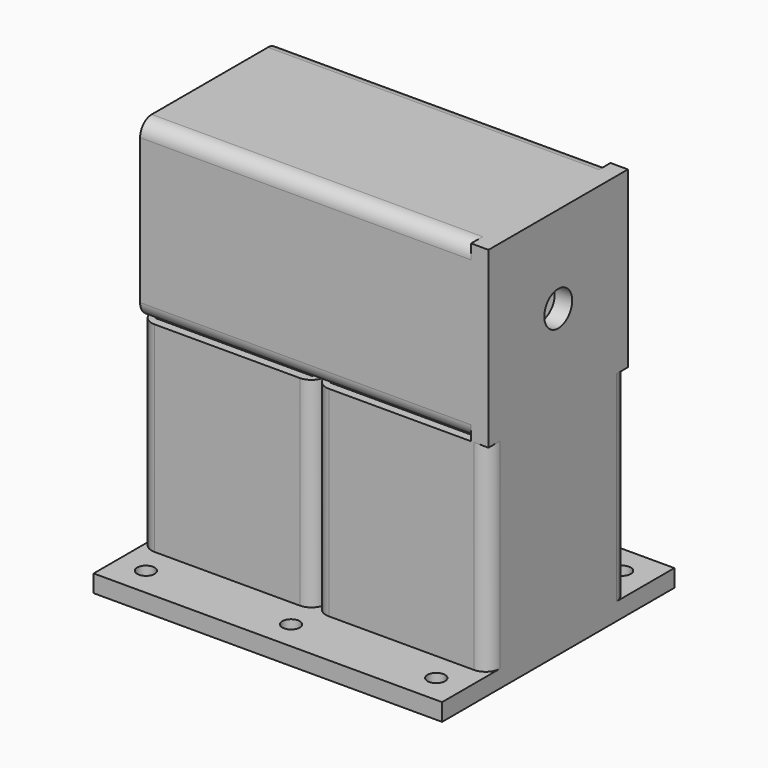
from build123d import *

# Parameters (mm, degrees)
F0_W     = 54
F0_H     = 54
F1_DEPTH = 69
F2_R     = 3
F2_W     = 54
F2_H     = 54
F3_DEPTH = 6
F4_W     = 54
F4_H     = 54
F5_DEPTH = 120
F6_W     = 60
F6_H     = 60
F6_R     = 6
F7_DEPTH = 6


with BuildPart() as f1:
    # F0 (on Top) → F1 (new body)
    with BuildSketch(Plane.XY):
        with BuildLine():
            ThreePointArc((-5.85040465, -3.5986092687), (-9.3859385559, -5.0630753627), (-10.85040465, -8.5986092687))
            Line((-10.85040465, -8.5986092687), (-10.85040465, -58.5986092687))
            ThreePointArc((-10.85040465, -58.5986092687), (-9.3859385559, -62.1341431746), (-5.85040465, -63.5986092687))
            Line((-5.85040465, -63.5986092687), (44.14959535, -63.5986092687))
            ThreePointArc((44.14959535, -63.5986092687), (47.685129256, -62.1341431746), (49.14959535, -58.5986092687))
            Line((49.14959535, -58.5986092687), (49.14959535, -8.5986092687))
            ThreePointArc((49.14959535, -8.5986092687), (47.685129256, -5.0630753627), (44.14959535, -3.5986092687))
            Line((44.14959535, -3.5986092687), (-5.85040465, -3.5986092687))
        make_face()
        with Locations((19.14959535, -33.5986092687)):
            Rectangle(F0_W, F0_H, mode=Mode.SUBTRACT)
        with BuildLine():
            ThreePointArc((54.14959535, -3.5986092687), (50.6140614441, -5.0630753627), (49.14959535, -8.5986092687))
            Line((49.14959535, -8.5986092687), (49.14959535, -58.5986092687))
            ThreePointArc((49.14959535, -58.5986092687), (50.6140614441, -62.1341431746), (54.14959535, -63.5986092687))
            Line((54.14959535, -63.5986092687), (104.14959535, -63.5986092687))
            ThreePointArc((104.14959535, -63.5986092687), (107.685129256, -62.1341431746), (109.14959535, -58.5986092687))
            Line((109.14959535, -58.5986092687), (109.14959535, -8.5986092687))
            ThreePointArc((109.14959535, -8.5986092687), (107.685129256, -5.0630753627), (104.14959535, -3.5986092687))
            Line((104.14959535, -3.5986092687), (54.14959535, -3.5986092687))
        make_face()
        with Locations((79.14959535, -33.5986092687)):
            Rectangle(F0_W, F0_H, mode=Mode.SUBTRACT)
    extrude(amount=F1_DEPTH)

    # F2 (on face) → F3 (join)
    with BuildSketch(Plane(origin=(0, 0, 0), x_dir=(1, 0, 0), z_dir=(0, 0, -1))):
        with BuildLine():
            Line((-10.85040465, -16.4013907313), (109.14959535, -16.4013907313))
            Line((109.14959535, -16.4013907313), (109.14959535, 8.5986092687))
            ThreePointArc((109.14959535, 8.5986092687), (107.685129256, 5.0630753627), (104.14959535, 3.5986092687))
            Line((104.14959535, 3.5986092687), (54.14959535, 3.5986092687))
            ThreePointArc((54.14959535, 3.5986092687), (50.6140614441, 5.0630753627), (49.14959535, 8.5986092687))
            ThreePointArc((49.14959535, 8.5986092687), (47.685129256, 5.0630753627), (44.14959535, 3.5986092687))
            Line((44.14959535, 3.5986092687), (-5.85040465, 3.5986092687))
            ThreePointArc((-5.85040465, 3.5986092687), (-9.3859385559, 5.0630753627), (-10.85040465, 8.5986092687))
            Line((-10.85040465, 8.5986092687), (-10.85040465, -16.4013907313))
        make_face()
        with Locations((-0.85040465, -6.4013907313)):
            Circle(F2_R, mode=Mode.SUBTRACT)
        with Locations((49.14959535, -6.4013907313)):
            Circle(F2_R, mode=Mode.SUBTRACT)
        with Locations((99.14959535, -6.4013907313)):
            Circle(F2_R, mode=Mode.SUBTRACT)
        with BuildLine():
            ThreePointArc((104.14959535, 63.5986092687), (107.685129256, 62.1341431746), (109.14959535, 58.5986092687))
            Line((109.14959535, 58.5986092687), (109.14959535, 83.5986092687))
            Line((109.14959535, 83.5986092687), (-10.85040465, 83.5986092687))
            Line((-10.85040465, 83.5986092687), (-10.85040465, 58.5986092687))
            ThreePointArc((-10.85040465, 58.5986092687), (-9.3859385559, 62.1341431746), (-5.85040465, 63.5986092687))
            Line((-5.85040465, 63.5986092687), (44.14959535, 63.5986092687))
            ThreePointArc((44.14959535, 63.5986092687), (47.685129256, 62.1341431746), (49.14959535, 58.5986092687))
            ThreePointArc((49.14959535, 58.5986092687), (50.6140614441, 62.1341431746), (54.14959535, 63.5986092687))
            Line((54.14959535, 63.5986092687), (104.14959535, 63.5986092687))
        make_face()
        with Locations((-0.85040465, 73.5986092687)):
            Circle(F2_R, mode=Mode.SUBTRACT)
        with Locations((49.14959535, 73.5986092687)):
            Circle(F2_R, mode=Mode.SUBTRACT)
        with Locations((99.14959535, 73.5986092687)):
            Circle(F2_R, mode=Mode.SUBTRACT)
        with BuildLine():
            ThreePointArc((104.14959535, 3.5986092687), (107.685129256, 5.0630753627), (109.14959535, 8.5986092687))
            Line((109.14959535, 8.5986092687), (109.14959535, 58.5986092687))
            ThreePointArc((109.14959535, 58.5986092687), (107.685129256, 62.1341431746), (104.14959535, 63.5986092687))
            Line((104.14959535, 63.5986092687), (54.14959535, 63.5986092687))
            ThreePointArc((54.14959535, 63.5986092687), (50.6140614441, 62.1341431746), (49.14959535, 58.5986092687))
            ThreePointArc((49.14959535, 58.5986092687), (47.685129256, 62.1341431746), (44.14959535, 63.5986092687))
            Line((44.14959535, 63.5986092687), (-5.85040465, 63.5986092687))
            ThreePointArc((-5.85040465, 63.5986092687), (-9.3859385559, 62.1341431746), (-10.85040465, 58.5986092687))
            Line((-10.85040465, 58.5986092687), (-10.85040465, 8.5986092687))
            ThreePointArc((-10.85040465, 8.5986092687), (-9.3859385559, 5.0630753627), (-5.85040465, 3.5986092687))
            Line((-5.85040465, 3.5986092687), (44.14959535, 3.5986092687))
            ThreePointArc((44.14959535, 3.5986092687), (47.685129256, 5.0630753627), (49.14959535, 8.5986092687))
            ThreePointArc((49.14959535, 8.5986092687), (50.6140614441, 5.0630753627), (54.14959535, 3.5986092687))
            Line((54.14959535, 3.5986092687), (104.14959535, 3.5986092687))
        make_face()
        with Locations((19.14959535, 33.5986092687)):
            Rectangle(F2_W, F2_H, mode=Mode.SUBTRACT)
        with Locations((79.14959535, 33.5986092687)):
            Rectangle(F2_W, F2_H, mode=Mode.SUBTRACT)
        with Locations((19.14959535, 33.5986092687)):
            Rectangle(F2_W, F2_H)
        with Locations((79.14959535, 33.5986092687)):
            Rectangle(F2_W, F2_H)
    extrude(amount=F3_DEPTH)

    # F4 (on face) → F5 (join, through all)
    with BuildSketch(Plane.YZ.offset(109.14959535)):
        with BuildLine():
            ThreePointArc((-3.5986092687, 124), (-5.0630753627, 127.5355339059), (-8.5986092687, 129))
            Line((-8.5986092687, 129), (-58.5986092687, 129))
            ThreePointArc((-58.5986092687, 129), (-62.1341431746, 127.5355339059), (-63.5986092687, 124))
            Line((-63.5986092687, 124), (-63.5986092687, 74))
            ThreePointArc((-63.5986092687, 74), (-62.1341431746, 70.4644660941), (-58.5986092687, 69))
            Line((-58.5986092687, 69), (-8.5986092687, 69))
            ThreePointArc((-8.5986092687, 69), (-5.0630753627, 70.4644660941), (-3.5986092687, 74))
            Line((-3.5986092687, 74), (-3.5986092687, 124))
        make_face()
        with Locations((-33.5986092687, 99)):
            Rectangle(F4_W, F4_H, mode=Mode.SUBTRACT)
    extrude(amount=-F5_DEPTH)

    # F6 (on face) → F7 (join)
    with BuildSketch(Plane.YZ.offset(109.14959535)):
        with Locations((-33.5986092687, 99)):
            Rectangle(F6_W, F6_H)
        with Locations((-33.5986092687, 99)):
            Circle(F6_R, mode=Mode.SUBTRACT)
    extrude(amount=-F7_DEPTH)


solid = f1.part
